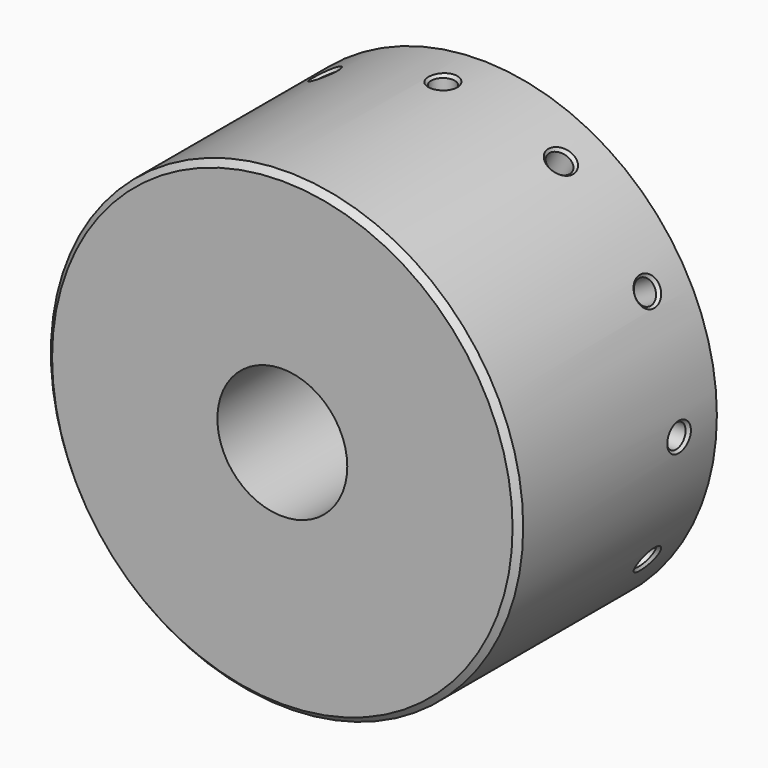
from build123d import *

# Parameters (mm, degrees)
F0_R            = 40
F1_DEPTH        = 42
F2_R            = 27.5
F3_DEPTH        = 3.5
F4_R            = 11
F5_DEPTH        = 105.4
F6_SIZE         = 1
F8_COPIES_COUNT = 12


# Not quite as in the source:
# - a pattern or mirror of a feature is missing from the dataset's text; its kind, count and spacing are read off the source's solid


with BuildPart() as f1:
    # F0 (on Front) → F1 (new body)
    with BuildSketch(Plane.XZ):
        Circle(F0_R)
    extrude(amount=F1_DEPTH)

    # F2 (on face) → F3 (cut)
    with BuildSketch(Plane(origin=(0, 0, 0), x_dir=(-1, 0, 0), z_dir=(0, 1, 0))):
        Circle(F2_R)
    extrude(amount=-F3_DEPTH, mode=Mode.SUBTRACT)

    # F4 (on face) → F5 (cut)
    with BuildSketch(Plane.XZ.offset(42)):
        Circle(F4_R)
    extrude(amount=-F5_DEPTH, mode=Mode.SUBTRACT)

    # F6
    f6_edges = [f1.edges().sort_by_distance(p)[0] for p in [
        (-40, -42, 0),
    ]]
    chamfer(f6_edges, length=F6_SIZE)

    # F7 (on Right) → F8 (revolve, cut)
    with BuildSketch(Plane.YZ):
        Polygon((-8, -35), (-8, -46.2057006681), (-6, -46.2057006681), (-4.9375298742, -40.5624701258), (-6, -39.5), (-6, -35), (-8, -34.0937713801), align=None)
    f8 = revolve(axis=Axis((0, -8, -40.6028503341), (0, 0, 1)), mode=Mode.SUBTRACT)

    # F8_copies: F8 ×12 about axis
    f8_copies_axis = Axis((0, 0, 0), (0, 1, 0))
    for i in range(1, F8_COPIES_COUNT):
        add(f8.rotate(f8_copies_axis, i * 360 / F8_COPIES_COUNT), mode=Mode.SUBTRACT)


solid = f1.part
